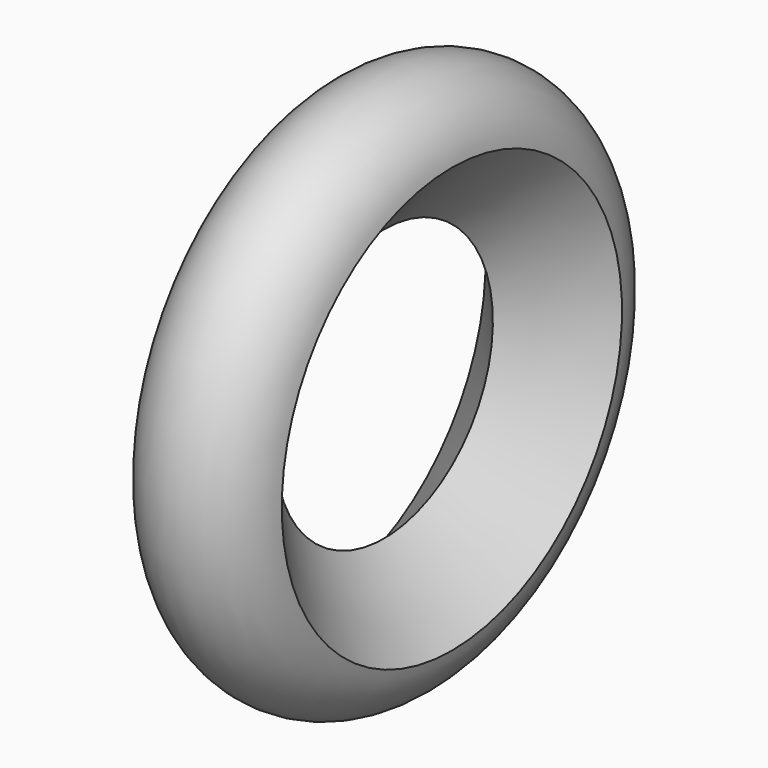
from build123d import *


# Not quite as in the source:
# - the program builds the solid bodies; features that only make, move or delete a surface that nothing else refers to are left out


with BuildPart() as f2:
    # F0 (on Front) → F2 (revolve)
    with BuildSketch(Plane.XZ):
        with BuildLine():
            ThreePointArc((15, 46.954241825), (-0.0704401471, 60.2114637334), (-15, 46.7957885154))
            Line((-15, 46.7957885154), (0, 30.0548467785))
            Line((0, 30.0548467785), (15, 46.954241825))
        make_face()
    revolve(axis=Axis((7.8298e-06, 0, 0), (1, 0, 0)))


solid = f2.part
